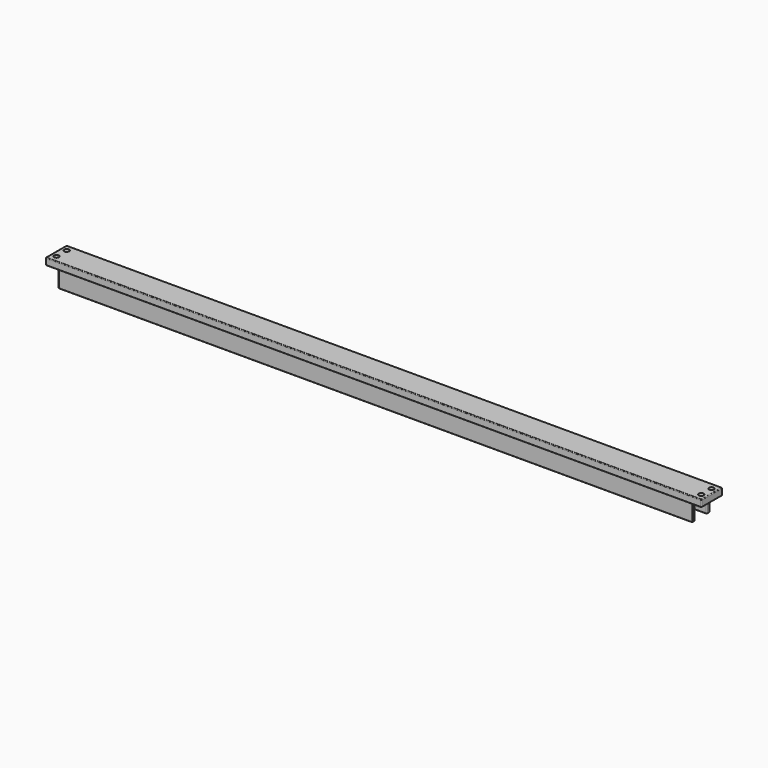
from build123d import *

# Parameters (mm, degrees)
F1_DEPTH = 465
F2_W     = 31
F2_H     = 25
F3_DEPTH = 15.5
F4_W     = 31
F4_H     = 25
F5_DEPTH = 15.5
F6_R     = 2
F7_DEPTH = 10.001
F8_R     = 3.5
F9_DEPTH = 4
F10_R    = 1
F11_R    = 1


# Not quite as in the source:
# - a pattern or mirror of a feature is missing from the dataset's text; its kind, count and spacing are read off the source's solid


with BuildPart() as f1:
    # F0 (on Right) → F1 (new body, symmetric)
    with BuildSketch(Plane.YZ):
        Polygon((18.5, 12.5), (-18.5, 12.5), (-18.5, 2.5), (-15.5, 2.5), (-15.5, -22.5), (-10.5, -22.5), (-10.5, 2.5), (0, 2.5), (10.5, 2.5), (10.5, -22.5), (15.5, -22.5), (15.5, 2.5), (18.5, 2.5), align=None)
    extrude(amount=F1_DEPTH, both=True)

    # F2 (on face) → F3 (cut)
    with BuildSketch(Plane(origin=(-465, 0, 0), x_dir=(0, -1, 0), z_dir=(-1, 0, 0))):
        with Locations((0, -10)):
            Rectangle(F2_W, F2_H)
    extrude(amount=-F3_DEPTH, mode=Mode.SUBTRACT)

    # F4 (on face) → F5 (cut)
    with BuildSketch(Plane.YZ.offset(465)):
        with Locations((0, -10)):
            Rectangle(F4_W, F4_H)
    extrude(amount=-F5_DEPTH, mode=Mode.SUBTRACT)

    # F6 (on face) → F7 (cut, through all)
    with BuildSketch(Plane(origin=(0, 0, 2.5), x_dir=(1, 0, 0), z_dir=(0, 0, -1))):
        with Locations((-457.25, 9)):
            Circle(F6_R)
        with Locations((-457.25, -9)):
            Circle(F6_R)
    f7 = extrude(amount=-F7_DEPTH, mode=Mode.SUBTRACT)

    # F7_copies: F7 across plane
    add(f7.mirror(Plane(origin=(0, 0, 0), x_dir=(0, 0, 1), z_dir=(1, 0, 0))), mode=Mode.SUBTRACT)

    # F8 (on face) → F9 (cut)
    with BuildSketch(Plane.XY.offset(12.5)):
        with Locations((-457.25, -9)):
            Circle(F8_R)
        with Locations((-457.25, 9)):
            Circle(F8_R)
    f9 = extrude(amount=-F9_DEPTH, mode=Mode.SUBTRACT)

    # F9_copies: F9 across plane
    add(f9.mirror(Plane(origin=(0, 0, 0), x_dir=(0, 0, 1), z_dir=(1, 0, 0))), mode=Mode.SUBTRACT)

    # F10
    f10_edges = [f1.edges().sort_by_distance(p)[0] for p in [
        (465, 18.5, 7.5),
        (465, -18.5, 7.5),
        (449.5, 13, -22.5),
        (449.5, -13, -22.5),
        (-465, -18.5, 7.5),
        (-449.5, -13, -22.5),
        (-449.5, 13, -22.5),
        (-465, 18.5, 7.5),
    ]]
    fillet(f10_edges, radius=F10_R)

    # F11
    f11_edges = [f1.edges().sort_by_distance(p)[0] for p in [
        (-449.5, -10.5, -9.5),
        (-449.5, -15.5, -9.5),
        (-449.5, 15.5, -9.5),
        (-449.5, 10.5, -9.5),
        (-449.5, 13, -21.5),
        (-449.5, 13, 2.5),
        (-465, 0, 2.5),
        (-465, 0, 12.5),
        (0, -15.5, 2.5),
        (-464.707107, 18.207107, 12.5),
        (-464.707107, -18.207107, 12.5),
        (0, 18.5, 12.5),
        (0, -18.5, 12.5),
        (464.707107, 18.207107, 12.5),
        (464.707107, -18.207107, 12.5),
        (465, 0, 12.5),
        (-464.707107, 18.207107, 2.5),
        (-464.707107, -18.207107, 2.5),
        (0, 18.5, 2.5),
        (0, -18.5, 2.5),
        (464.707107, 18.207107, 2.5),
        (464.707107, -18.207107, 2.5),
        (465, 0, 2.5),
        (-449.5, -13, 2.5),
        (449.5, -13, 2.5),
        (0, -10.5, 2.5),
        (0, 10.5, 2.5),
        (449.5, 13, 2.5),
        (0, 15.5, 2.5),
        (449.5, -15.5, -9.5),
        (449.207107, -15.5, -22.207107),
        (0, -15.5, -22.5),
        (-449.207107, -15.5, -22.207107),
        (449.5, -10.5, -9.5),
        (0, -10.5, -22.5),
        (-449.207107, -10.5, -22.207107),
        (449.207107, -10.5, -22.207107),
        (449.5, 10.5, -9.5),
        (449.207107, 10.5, -22.207107),
        (0, 10.5, -22.5),
        (-449.207107, 10.5, -22.207107),
        (449.5, 15.5, -9.5),
        (0, 15.5, -22.5),
        (-449.207107, 15.5, -22.207107),
        (449.207107, 15.5, -22.207107),
    ]]
    fillet(f11_edges, radius=F11_R)


solid = f1.part
